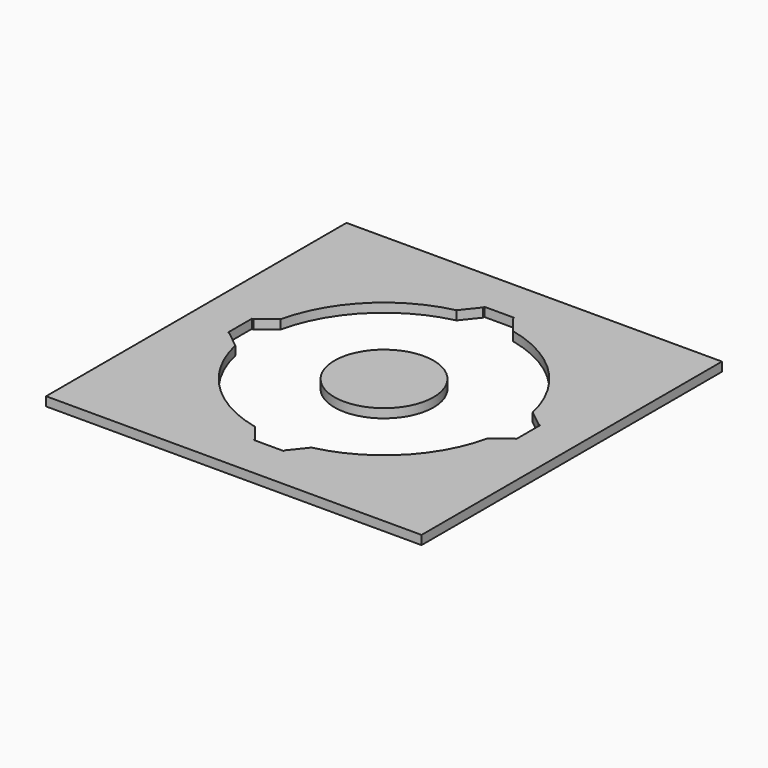
from build123d import *

# Parameters (mm, degrees)
F0_W        = 500
F0_H        = 500
F1_DEPTH    = 12
F2_R        = 66
F3_DEPTH    = 12
F4_T1_DEPTH = 111.3908314838


# Not quite as in the source:
# - a fillet or chamfer that OpenCascade refuses, or shapes differently, is made with other operations: its cross-section is extruded or revolved along the edge and cut away or added


with BuildPart() as f1:
    # F0 (on Top) → F1 (new body)
    with BuildSketch(Plane.XY):
        Rectangle(F0_W, F0_H)
    extrude(amount=F1_DEPTH)

    # F2 (on face) → F3 (cut, through all)
    with BuildSketch(Plane(origin=(0, 0, 0), x_dir=(1, 0, 0), z_dir=(0, 0, -1))):
        with BuildLine():
            ThreePointArc((170.8332520325, -20), (171.7080652584, -10.0170018072), (172, 0))
            ThreePointArc((172, 0), (171.7080652584, 10.0170018072), (170.8332520325, 20))
            ThreePointArc((170.8332520325, 20), (121.6223663641, 121.6223663641), (20, 170.8332520325))
            ThreePointArc((20, 170.8332520325), (0, 172), (-20, 170.8332520325))
            ThreePointArc((-20, 170.8332520325), (-121.6223663641, 121.6223663641), (-170.8332520325, 20))
            ThreePointArc((-170.8332520325, 20), (-172, 0), (-170.8332520325, -20))
            ThreePointArc((-170.8332520325, -20), (-121.6223663641, -121.6223663641), (-20, -170.8332520325))
            ThreePointArc((-20, -170.8332520325), (0, -172), (20, -170.8332520325))
            ThreePointArc((20, -170.8332520325), (121.6223663641, -121.6223663641), (170.8332520325, -20))
        make_face()
        Circle(F2_R, mode=Mode.SUBTRACT)
        with BuildLine():
            ThreePointArc((170.8332520325, 20), (171.7080652584, 10.0170018072), (172, 0))
            ThreePointArc((172, 0), (171.7080652584, -10.0170018072), (170.8332520325, -20))
            Line((170.8332520325, -20), (192, -20))
            Line((192, -20), (192, 20))
            Line((192, 20), (170.8332520325, 20))
        make_face()
        with BuildLine():
            ThreePointArc((-20, 170.8332520325), (0, 172), (20, 170.8332520325))
            Line((20, 170.8332520325), (20, 192))
            Line((20, 192), (-20, 192))
            Line((-20, 192), (-20, 170.8332520325))
        make_face()
        with BuildLine():
            Line((20, -192), (20, -170.8332520325))
            ThreePointArc((20, -170.8332520325), (0, -172), (-20, -170.8332520325))
            Line((-20, -170.8332520325), (-20, -192))
            Line((-20, -192), (20, -192))
        make_face()
        with BuildLine():
            ThreePointArc((-170.8332520325, -20), (-172, 0), (-170.8332520325, 20))
            Line((-170.8332520325, 20), (-192, 20))
            Line((-192, 20), (-192, -20))
            Line((-192, -20), (-170.8332520325, -20))
        make_face()
    extrude(amount=-F3_DEPTH, mode=Mode.SUBTRACT)

    # F4: chamfer of 20.32 on 8 edges, made by hand

    # F4_s2 → F4_t1 (cut)
    with BuildSketch(Plane.XY.offset(-49.6954157419)):
        with BuildLine():
            Line((-167.1564879531, 38.3241668303), (-190.7049353821, 19.4923621634))
            Line((-190.7049353821, 19.4923621634), (-190.7049353821, 19.0859621634))
            ThreePointArc((-190.7049353821, 19.0859621634), (-180.7690937073, 19.5936), (-170.8332520325, 19.5936))
            Line((-170.8332520325, 19.5936), (-170.4296088137, 19.952744186))
            ThreePointArc((-170.4296088137, 19.952744186), (-169.0944526119, 29.1792675855), (-166.7600323023, 38.2348142873))
            Line((-166.7600323023, 38.2348142873), (-167.1564879531, 38.3241668303))
        make_face()
        with BuildLine():
            Line((-190.7049353821, -19.4923621634), (-167.1564879531, -38.3241668303))
            Line((-167.1564879531, -38.3241668303), (-166.7600323023, -38.2348142873))
            ThreePointArc((-166.7600323023, -38.2348142873), (-169.0944526119, -29.1792675855), (-170.4296088137, -19.952744186))
            Line((-170.4296088137, -19.952744186), (-170.8332520325, -19.5936))
            ThreePointArc((-170.8332520325, -19.5936), (-180.7690937073, -19.5936), (-190.7049353821, -19.0859621634))
            Line((-190.7049353821, -19.0859621634), (-190.7049353821, -19.4923621634))
        make_face()
        with BuildLine():
            Line((-38.3241668303, -167.1564879531), (-19.4923621634, -190.7049353821))
            Line((-19.4923621634, -190.7049353821), (-19.0859621634, -190.7049353821))
            ThreePointArc((-19.0859621634, -190.7049353821), (-19.5936, -180.7690937073), (-19.5936, -170.8332520325))
            Line((-19.5936, -170.8332520325), (-19.952744186, -170.4296088137))
            ThreePointArc((-19.952744186, -170.4296088137), (-29.1792675855, -169.0944526119), (-38.2348142873, -166.7600323023))
            Line((-38.2348142873, -166.7600323023), (-38.3241668303, -167.1564879531))
        make_face()
        with BuildLine():
            Line((19.4923621634, -190.7049353821), (38.3241668303, -167.1564879531))
            Line((38.3241668303, -167.1564879531), (38.2348142873, -166.7600323023))
            ThreePointArc((38.2348142873, -166.7600323023), (29.1792675855, -169.0944526119), (19.952744186, -170.4296088137))
            Line((19.952744186, -170.4296088137), (19.5936, -170.8332520325))
            ThreePointArc((19.5936, -170.8332520325), (19.5936, -180.7690937073), (19.0859621634, -190.7049353821))
            Line((19.0859621634, -190.7049353821), (19.4923621634, -190.7049353821))
        make_face()
        with BuildLine():
            Line((190.7049353821, 19.4923621634), (167.1564879531, 38.3241668303))
            Line((167.1564879531, 38.3241668303), (166.7600323023, 38.2348142873))
            ThreePointArc((166.7600323023, 38.2348142873), (169.0944526119, 29.1792675855), (170.4296088137, 19.952744186))
            Line((170.4296088137, 19.952744186), (170.8332520325, 19.5936))
            ThreePointArc((170.8332520325, 19.5936), (180.7690937073, 19.5936), (190.7049353821, 19.0859621634))
            Line((190.7049353821, 19.0859621634), (190.7049353821, 19.4923621634))
        make_face()
        with BuildLine():
            Line((-19.4923621634, 190.7049353821), (-38.3241668303, 167.1564879531))
            Line((-38.3241668303, 167.1564879531), (-38.2348142873, 166.7600323023))
            ThreePointArc((-38.2348142873, 166.7600323023), (-29.1792675855, 169.0944526119), (-19.952744186, 170.4296088137))
            Line((-19.952744186, 170.4296088137), (-19.5936, 170.8332520325))
            ThreePointArc((-19.5936, 170.8332520325), (-19.5936, 180.7690937073), (-19.0859621634, 190.7049353821))
            Line((-19.0859621634, 190.7049353821), (-19.4923621634, 190.7049353821))
        make_face()
        with BuildLine():
            Line((38.3241668303, 167.1564879531), (19.4923621634, 190.7049353821))
            Line((19.4923621634, 190.7049353821), (19.0859621634, 190.7049353821))
            ThreePointArc((19.0859621634, 190.7049353821), (19.5936, 180.7690937073), (19.5936, 170.8332520325))
            Line((19.5936, 170.8332520325), (19.952744186, 170.4296088137))
            ThreePointArc((19.952744186, 170.4296088137), (29.1792675855, 169.0944526119), (38.2348142873, 166.7600323023))
            Line((38.2348142873, 166.7600323023), (38.3241668303, 167.1564879531))
        make_face()
        with BuildLine():
            Line((190.7049353821, -19.4923621634), (167.1564879531, -38.3241668303))
            Line((167.1564879531, -38.3241668303), (166.7600323023, -38.2348142873))
            ThreePointArc((166.7600323023, -38.2348142873), (169.0944526119, -29.1792675855), (170.4296088137, -19.952744186))
            Line((170.4296088137, -19.952744186), (170.8332520325, -19.5936))
            ThreePointArc((170.8332520325, -19.5936), (180.7690937073, -19.5936), (190.7049353821, -19.0859621634))
            Line((190.7049353821, -19.0859621634), (190.7049353821, -19.4923621634))
        make_face()
    extrude(amount=F4_T1_DEPTH, mode=Mode.SUBTRACT)


solid = f1.part
